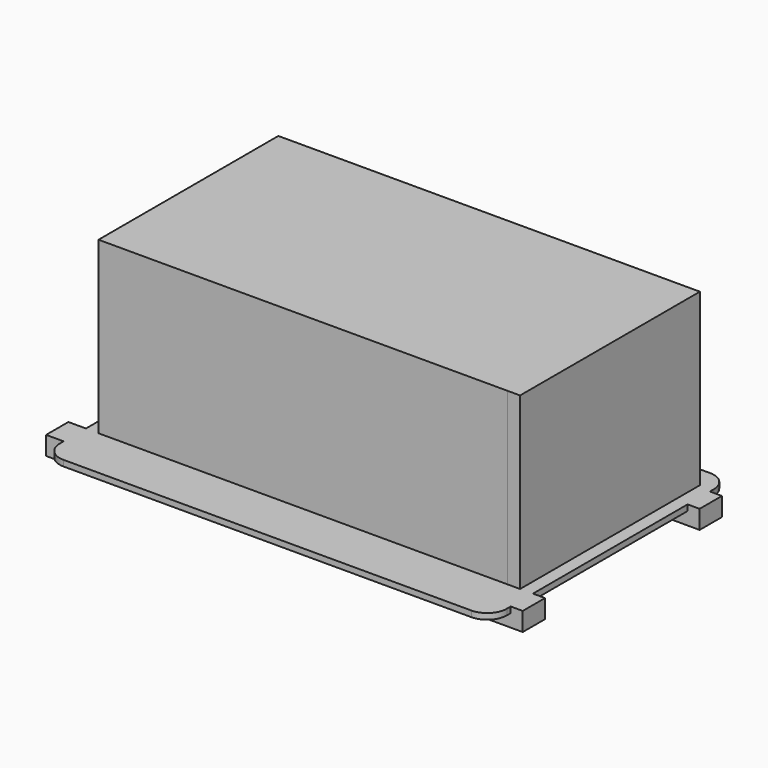
from build123d import *

# Parameters (mm, degrees)
F0_W     = 123.629912734
F0_H     = 7.2298198938
F1_DEPTH = 4.826
F2_W     = 115.9501895308
F2_H     = 7.2298198938
F2_H_2   = 6.35
F2_H_3   = 63.7065680534
F3_DEPTH = 1.524
F5_R     = 5.08
F6_W     = 102.7462986398
F6_H     = 3.4007430077
F6_H_2   = 3.4007552
F7_DEPTH = 44.196
F8_DEPTH = 44.196


# Not quite as in the source:
# - ends of sketch curves that miss each other by under 0.0002 mm in the source are joined


with BuildPart() as f1:
    # F0 (on Top) → F1 (new body)
    with BuildSketch(Plane.XY):
        with Locations((-2.2894367576, -16.3875911385)):
            Rectangle(F0_W, F0_H)
    extrude(amount=F1_DEPTH)


with BuildPart() as f1b:
    # F0 (on Top) → F1, piece 2 (new body)
    with BuildSketch(Plane.XY):
        with Locations((-2.2894367576, 40.9689769149)):
            Rectangle(F0_W, F0_H)
    extrude(amount=F1_DEPTH)


with BuildPart() as f3:
    # F2 (on face) → F3 (new body)
    with BuildSketch(Plane.XY.offset(4.826)):
        with Locations((-1.5743747354, 40.9689769149)):
            Rectangle(F2_W, F2_H)
        with Locations((-1.5743747354, 47.7588868618)):
            Rectangle(F2_W, F2_H_2)
        with Locations((-1.5743747354, 5.5007829413)):
            Rectangle(F2_W, F2_H_3)
    extrude(amount=-F3_DEPTH)


with BuildPart() as f1b_1:
    add(f1b.part)

    # F4: union F3, F1
    add(f3.part)
    add(f1.part)

    # F5
    f5_edges = [f1b_1.edges().sort_by_distance(p)[0] for p in [
        (-59.54947, -26.352501, 4.064),
        (56.40072, -26.352501, 4.064),
        (56.40072, 50.933887, 4.064),
        (-59.54947, 50.933887, 4.064),
    ]]
    fillet(f5_edges, radius=F5_R)

    # F6 (on face) → F7 (join)
    with BuildSketch(Plane.XY.offset(4.826)):
        Polygon((-52.9475212097, 45.4720444977), (-56.2473237514, 45.4720444977), (-56.2473237514, -12.8244720399), (-52.9475212097, -12.8244720399), (-52.9475212097, -9.4237168399), (-52.9475212097, 42.0713014901), align=None)
        with Locations((-1.5743718898, 43.7716729939)):
            Rectangle(F6_W, F6_H)
        Polygon((53.0985676301, 45.4720334084), (49.7987774301, 45.4720334084), (49.7987774301, 42.0713014901), (49.7987774301, -9.4237168399), (49.7987774301, -12.8244717916), (53.0985676301, -12.8244717916), align=None)
        with Locations((-1.5743718898, -11.1240944399)):
            Rectangle(F6_W, F6_H_2)
    extrude(amount=F7_DEPTH)

    # F8 (add): a face of the model
    f8_faces = [f1b_1.faces().sort_by_distance(p)[0] for p in [
        (-1.5743718898, 16.3237923251, 4.826),
    ]]
    extrude(f8_faces, amount=F8_DEPTH)


solid = f1b_1.part
